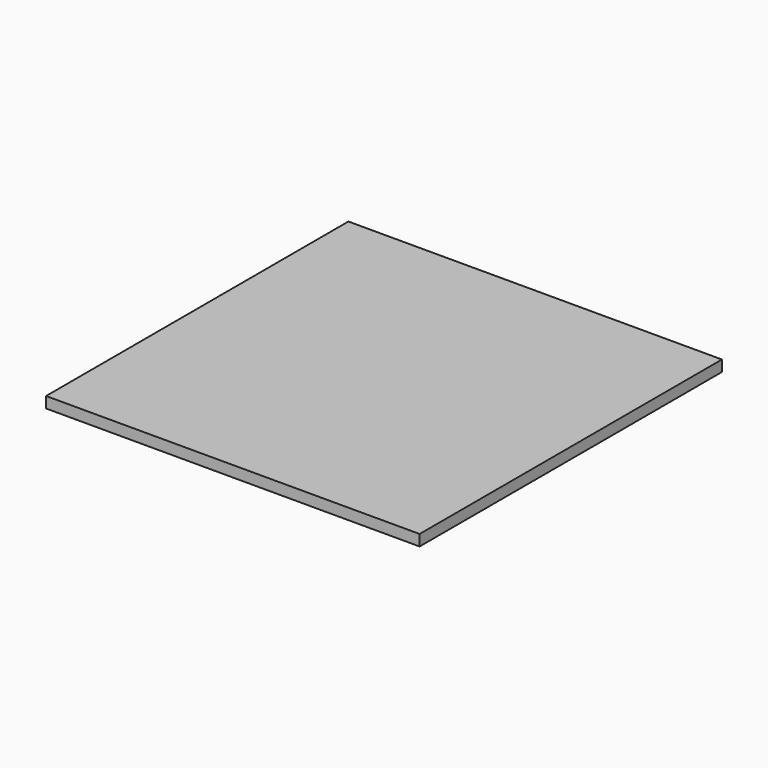
from build123d import *

# Parameters (mm, degrees)
F0_W     = 215.1707336307
F0_H     = 217.666676268
F1_DEPTH = 6.35


# Not quite as in the source:
# - the program builds the solid bodies; features that only make, move or delete a surface that nothing else refers to are left out


with BuildPart() as f1:
    # F0 (on Top) → F1 (new body)
    with BuildSketch(Plane.XY):
        with Locations((6.2649138272, 19.6214737371)):
            Rectangle(F0_W, F0_H)
    extrude(amount=F1_DEPTH)


solid = f1.part
